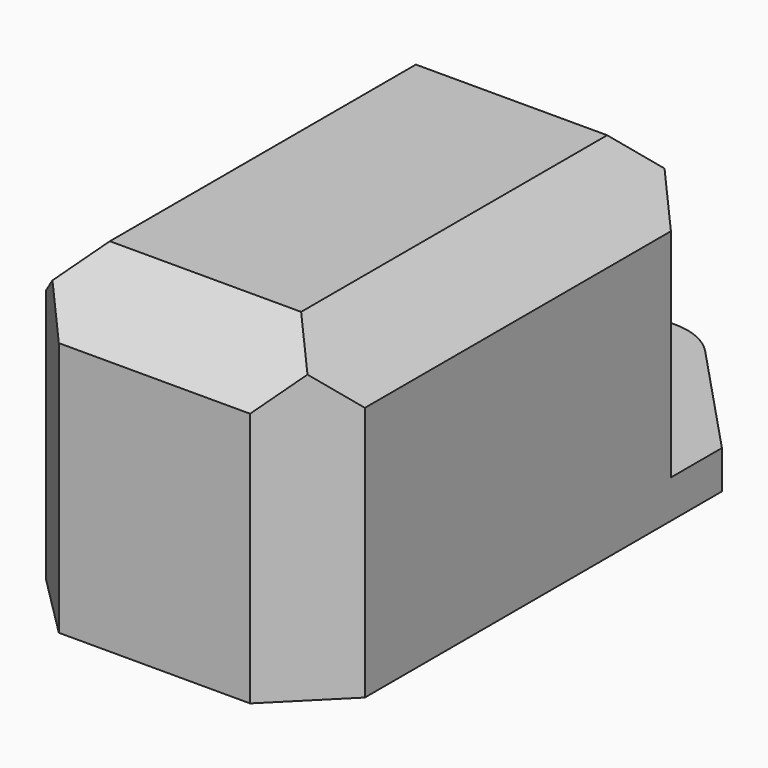
from build123d import *

# Parameters (mm, degrees)
F0_W        = 25
F0_H        = 40
F1_DEPTH    = 25
F0_R        = 2
F2_DEPTH    = 3
F3_SIZE     = 5
F4_SIZE     = 5
F5_T        = 3
F5_T3_DEPTH = 21
F5_T5_DEPTH = 13.0710678119
F5_T7_DEPTH = 13.0710678119


# Not quite as in the source:
# - a shell that OpenCascade refuses in one call is made with other operations: the cavity is built on its own and cut out


with BuildPart() as f1:
    # F0 (on Top) → F1 (new body)
    with BuildSketch(Plane.XY):
        Rectangle(F0_W, F0_H)
    extrude(amount=F1_DEPTH)

    # F0 (on Top) → F2 (join)
    with BuildSketch(Plane.XY):
        with BuildLine():
            Line((-3.6435657461, 29.4240953044), (-12.5, 20))
            Line((-12.5, 20), (12.5, 20))
            Line((12.5, 20), (3.6435657461, 29.4240953044))
            ThreePointArc((3.6435657461, 29.4240953044), (4.6485389495, 27.8414900583), (5, 26))
            ThreePointArc((5, 26), (-1.8414900583, 21.3514610505), (-3.6435657461, 29.4240953044))
        make_face()
        with BuildLine():
            ThreePointArc((3.6435657461, 29.4240953044), (0, 31), (-3.6435657461, 29.4240953044))
            ThreePointArc((-3.6435657461, 29.4240953044), (-1.8414900583, 21.3514610505), (5, 26))
            ThreePointArc((5, 26), (4.6485389495, 27.8414900583), (3.6435657461, 29.4240953044))
        make_face()
        with Locations((0, 26)):
            Circle(F0_R, mode=Mode.SUBTRACT)
    extrude(amount=F2_DEPTH)

    # F3
    f3_edges = [f1.edges().sort_by_distance(p)[0] for p in [
        (12.5, 0, 25),
        (0, -20, 25),
        (-12.5, 0, 25),
        (0, 20, 25),
    ]]
    chamfer(f3_edges, length=F3_SIZE)

    # F4
    f4_edges = [f1.edges().sort_by_distance(p)[0] for p in [
        (-12.5, -20, 10),
        (12.5, -20, 10),
        (12.5, 20, 11.5),
        (-12.5, 20, 11.5),
    ]]
    chamfer(f4_edges, length=F4_SIZE)

    # F5: shell of thickness 3, made by hand


with BuildPart() as f5_core1:
    # F5_t2: copy of F1
    add(f1.part)

    # the walls: a layer under each face that stays
    f5_faces = [f5_core1.faces().sort_by_distance(p)[0] for p in [
        (0, 20, 11.5),
        (0, 17.5, 22.5),
        (10, 17.5, 12.75),
        (-10, 17.5, 12.75),
        (0, 23, 3),
        (10, 0, 22.5),
        (0, 0, 25),
        (-10, 0, 22.5),
        (12.5, 2.5, 10),
        (-12.5, 2.5, 10),
        (-8.0717828731, 24.7120476522, 1.5),
        (8.0717828731, 24.7120476522, 1.5),
        (0, 31, 1.5),
        (-2, 26, 1.5),
        (0, -17.5, 22.5),
        (10, -17.5, 11.25),
        (-10, -17.5, 11.25),
        (0, -20, 10),
    ]]
    thicken(f5_faces, amount=-F5_T, mode=Mode.SUBTRACT)

    # F5_s4 → F5_t3 (cut)
    with BuildSketch(Plane.YZ.offset(-10.5)):
        Polygon((20.03, 3.03), (17, 3), (17, 0), (20, 0), align=None)
    extrude(amount=F5_T3_DEPTH, mode=Mode.SUBTRACT)

    # F5_s6 → F5_t5 (cut)
    with BuildSketch(Plane(origin=(-8.3713203436, 8.3713203436, 0), x_dir=(0, 0, 1), z_dir=(0.7071067812, -0.7071067812, 0))):
        Polygon((3.03, -19.4754364826), (3, -16.4454364826), (0, -16.4454364826), (0, -19.4454364826), align=None)
    extrude(amount=F5_T5_DEPTH, mode=Mode.SUBTRACT)

    # F5_s8 → F5_t7 (cut)
    with BuildSketch(Plane(origin=(8.3713203436, 8.3713203436, 0), x_dir=(0, 0, 1), z_dir=(-0.7071067812, -0.7071067812, 0))):
        Polygon((3.03, 19.4754364826), (3, 16.4454364826), (0, 16.4454364826), (0, 19.4454364826), align=None)
    extrude(amount=F5_T7_DEPTH, mode=Mode.SUBTRACT)


with BuildPart() as f1_1:
    add(f1.part)

    # what is left inside the walls is the cavity
    f5_cavity = [f5_core1.part.solids().sort_by_distance(p)[0] for p in [
        (0, -5.666667, 0.03),
    ]]
    add(f5_cavity, mode=Mode.SUBTRACT)


solid = f1_1.part
